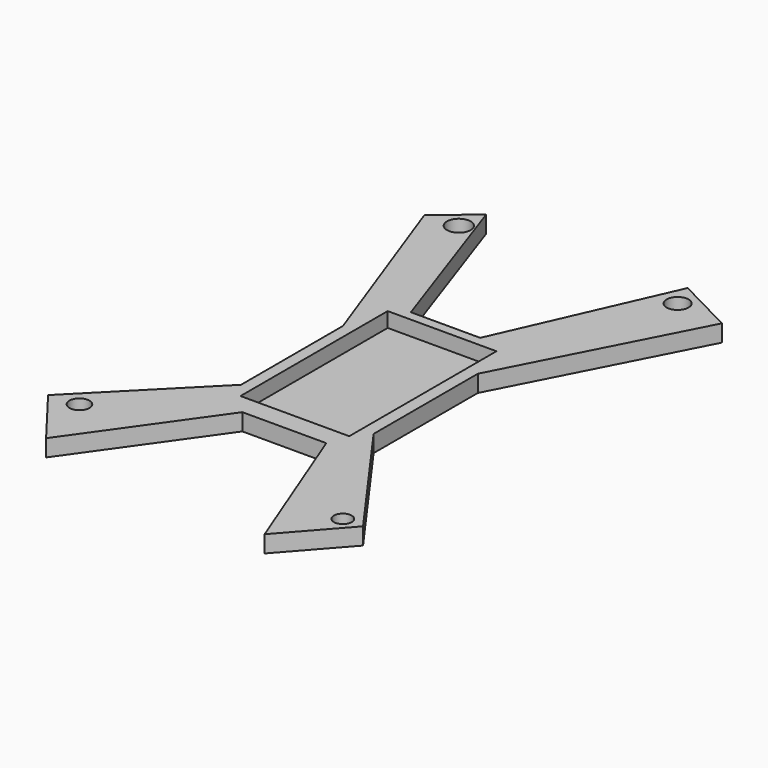
from build123d import *

# Parameters (mm, degrees)
F0_W     = 39.0892345458
F0_H     = 66.1229081452
F1_DEPTH = 0.762
F0_R     = 4.2603265816
F0_R_2   = 3.9515412254
F0_R_3   = 3.5979856565
F0_R_4   = 3.2023821092
F2_DEPTH = 6.096


# Not quite as in the source:
# - a feature of the source that left no trace in its solid (it failed there, or was rolled back) is left out


with BuildPart() as f1:
    # F0 (on Top) → F1 (new body)
    with BuildSketch(Plane.XY):
        with Locations((2.9225489125, -2.8168093413)):
            Rectangle(F0_W, F0_H)
    extrude(amount=F1_DEPTH)

    # F0 (on Top) → F2 (join)
    with BuildSketch(Plane.XY):
        Polygon((-20.7744576037, 15.3352888301), (-20.7744576037, 33.758495003), (-11.104892008, 33.758495003), (-31.6940061748, 93.3202803135), (-45.0146831572, 82.2209268808), align=None)
        with Locations((-33.4267839789, 83.2160338759)):
            Circle(F0_R, mode=Mode.SUBTRACT)
        Polygon((-11.104892008, 33.758495003), (-20.7744576037, 33.758495003), (-20.7744576037, 15.3352888301), (-20.7744576037, -30.4260663688), (-20.7744576037, -43.2014353573), (-10.0806253031, -43.2014353573), (20.0740266591, -43.2014353573), (26.9123706967, -43.2014353573), (26.9123706967, -30.5006168783), (26.9123706967, 16.304789111), (26.9123706967, 33.758495003), (13.8152288273, 33.758495003), align=None)
        with Locations((2.9225489125, -2.8168093413)):
            Rectangle(F0_W, F0_H, mode=Mode.SUBTRACT)
        Polygon((40.3667656029, 93.7842203212), (13.8152288273, 33.758495003), (26.9123706967, 33.758495003), (26.9123706967, 16.304789111), (61.2783841789, 83.0108523369), align=None)
        with Locations((44.0210402012, 84.6773162484)):
            Circle(F0_R_2, mode=Mode.SUBTRACT)
        Polygon((-20.7744576037, -43.2014353573), (-20.7744576037, -30.4260663688), (-59.1404661536, -69.1590458155), (-43.2117395103, -89.9672359228), (-10.0806253031, -43.2014353573), align=None)
        with Locations((-48.7702228129, -68.0264160037)):
            Circle(F0_R_3, mode=Mode.SUBTRACT)
        Polygon((59.6924833953, -76.2155726552), (26.9123706967, -30.5006168783), (26.9123706967, -43.2014353573), (20.0740266591, -43.2014353573), (41.1184616387, -97.2259193659), align=None)
        with Locations((52.4233952165, -76.2155726552)):
            Circle(F0_R_4, mode=Mode.SUBTRACT)
    extrude(amount=F2_DEPTH)


solid = f1.part
